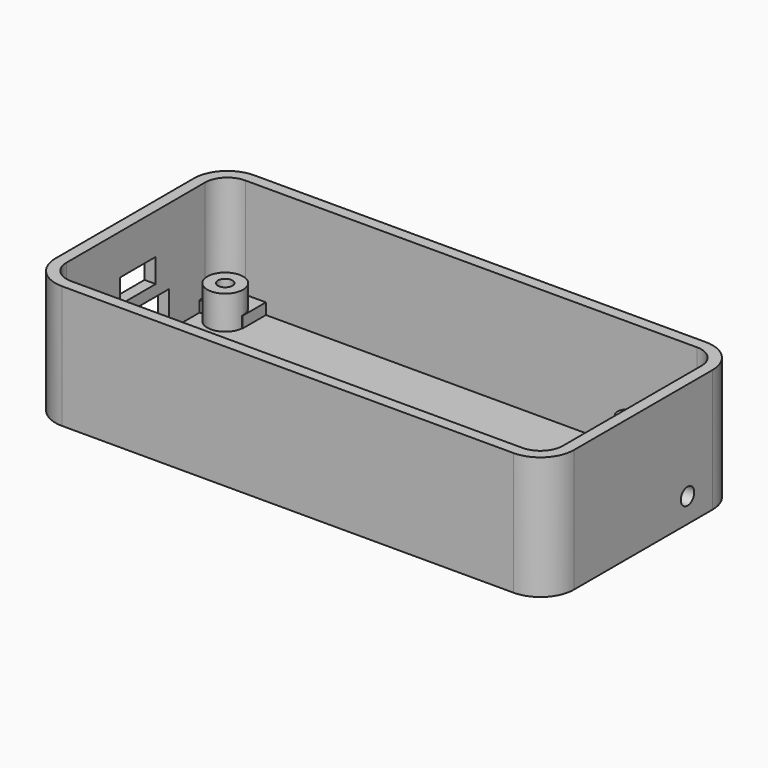
from build123d import *

# Parameters (mm, degrees)
F1_DEPTH  = 13.97
F2_T      = -1.27
F3_R      = 2.032
F3_R_2    = 0.8255
F4_DEPTH  = 3.81
F5_DEPTH  = 5.461
F6_DEPTH  = 2.54
F7_W      = 8.89
F7_H      = 3.1753103511
F7_W_2    = 5.08
F7_H_2    = 2.7178
F8_DEPTH  = 1.905
F9_R      = 0.9525
F10_DEPTH = 1.905
F11_R     = 2.032
F11_R_2   = 0.8255
F12_DEPTH = 3.81
F14_DEPTH = 2.032
F15_W     = 3.3083129674
F15_H     = 4.001185298
F15_W_2   = 4.9948431551
F15_H_2   = 3.4223934636
F15_W_3   = 4.9023460597
F15_H_3   = 4.0236227214
F16_DEPTH = 1.27


with BuildPart() as f1:
    # F0 (on Top) → F1 (new body)
    with BuildSketch(Plane.XY):
        with BuildLine():
            Line((-21.5788040441, -13.9683183577), (29.7179990722, -13.9683183577))
            ThreePointArc((29.7179990722, -13.9683183577), (32.4120759085, -12.852395194), (33.5279990722, -10.1583183577))
            Line((33.5279990722, -10.1583183577), (33.5279990722, 9.5266816423))
            ThreePointArc((33.5279990722, 9.5266816423), (32.4120759085, 12.2207584786), (29.7179990722, 13.3366816423))
            Line((29.7179990722, 13.3366816423), (-21.60052527, 13.3366816423))
            ThreePointArc((-21.60052527, 13.3366816423), (-24.2960880723, 12.2192716925), (-25.4105229505, 9.5224775366))
            Line((-25.4105229505, 9.5224775366), (-25.3888017246, -10.1625224634))
            ThreePointArc((-25.3888017246, -10.1625224634), (-24.2713940943, -12.8538811601), (-21.5788040441, -13.9683183577))
        make_face()
    extrude(amount=F1_DEPTH)

    # F2
    f2_openings = [f1.faces().sort_by_distance(p)[0] for p in [
        (4.064166, -0.31477, 13.97),
    ]]
    offset(amount=F2_T, openings=f2_openings)

    # F3 (on face) → F4 (join)
    with BuildSketch(Plane.XY.offset(1.27)):
        with Locations((-21.3360009278, 8.8916816423)):
            Circle(F3_R)
        with Locations((-21.3360009278, 8.8916816423)):
            Circle(F3_R_2, mode=Mode.SUBTRACT)
        with Locations((-21.3360009278, -8.8883183577)):
            Circle(F3_R)
        with Locations((-21.3360009278, -8.8883183577)):
            Circle(F3_R_2, mode=Mode.SUBTRACT)
        with BuildLine():
            Line((26.9239990722, -8.8883183577), (25.5269990722, -8.8883183577))
            ThreePointArc((25.5269990722, -8.8883183577), (24.3839990722, -10.0313183577), (23.2409990722, -8.8883183577))
            Line((23.2409990722, -8.8883183577), (21.8439990722, -8.8883183577))
            ThreePointArc((21.8439990722, -8.8883183577), (24.3839990722, -11.4283183577), (26.9239990722, -8.8883183577))
        make_face()
        with BuildLine():
            ThreePointArc((23.2409990722, 8.8916816423), (24.3839990722, 10.0346816423), (25.5269990722, 8.8916816423))
            Line((25.5269990722, 8.8916816423), (26.9239990722, 8.8916816423))
            ThreePointArc((26.9239990722, 8.8916816423), (24.3839990722, 11.4316816423), (21.8439990722, 8.8916816423))
            Line((21.8439990722, 8.8916816423), (23.2409990722, 8.8916816423))
        make_face()
    extrude(amount=F4_DEPTH)

    # F3 (on face) → F5 (join)
    with BuildSketch(Plane.XY.offset(1.27)):
        with BuildLine():
            Line((24.3839990722, 8.8916816423), (25.5269990722, 8.8916816423))
            ThreePointArc((25.5269990722, 8.8916816423), (24.3839990722, 10.0346816423), (23.2409990722, 8.8916816423))
            Line((23.2409990722, 8.8916816423), (24.3839990722, 8.8916816423))
        make_face()
        with BuildLine():
            ThreePointArc((23.2409990722, 8.8916816423), (24.3839990722, 7.7486816423), (25.5269990722, 8.8916816423))
            Line((25.5269990722, 8.8916816423), (24.3839990722, 8.8916816423))
            Line((24.3839990722, 8.8916816423), (23.2409990722, 8.8916816423))
        make_face()
        with BuildLine():
            Line((24.3839990722, -8.8883183577), (25.5269990722, -8.8883183577))
            ThreePointArc((25.5269990722, -8.8883183577), (24.3839990722, -7.7453183577), (23.2409990722, -8.8883183577))
            Line((23.2409990722, -8.8883183577), (24.3839990722, -8.8883183577))
        make_face()
        with BuildLine():
            ThreePointArc((23.2409990722, -8.8883183577), (24.3839990722, -10.0313183577), (25.5269990722, -8.8883183577))
            Line((25.5269990722, -8.8883183577), (24.3839990722, -8.8883183577))
            Line((24.3839990722, -8.8883183577), (23.2409990722, -8.8883183577))
        make_face()
    extrude(amount=F5_DEPTH)

    # F3 (on face) → F6 (cut)
    with BuildSketch(Plane.XY.offset(1.27)):
        with Locations((-21.3360009278, 8.8916816423)):
            Circle(F3_R_2)
        with Locations((-21.3360009278, -8.8883183577)):
            Circle(F3_R_2)
    extrude(amount=F6_DEPTH, mode=Mode.SUBTRACT)

    # F7 (on face) → F8 (cut)
    with BuildSketch(Plane(origin=(-25.3999845367, -0.0280273712, 0), x_dir=(0.0011034398, -0.9999993912, 0), z_dir=(-0.9999993912, -0.0011034398, 0))):
        with Locations((0, 3.81)):
            Rectangle(F7_W, F7_H)
        with Locations((0, 8.0265551756)):
            Rectangle(F7_W_2, F7_H_2)
    extrude(amount=-F8_DEPTH, mode=Mode.SUBTRACT)

    # F9 (on face) → F10 (cut)
    with BuildSketch(Plane.YZ.offset(33.5279990722)):
        with Locations((5.9706816423, 2.794)):
            Circle(F9_R)
    extrude(amount=-F10_DEPTH, mode=Mode.SUBTRACT)

    # F11 (on face) → F12 (join)
    with BuildSketch(Plane.XY.offset(1.27)):
        with Locations((29.4639990722, 0)):
            Circle(F11_R)
        with Locations((29.4639990722, 0)):
            Circle(F11_R_2, mode=Mode.SUBTRACT)
    extrude(amount=F12_DEPTH)

    # F13 (on face) → F14 (join)
    with BuildSketch(Plane.XY.offset(1.27)):
        with BuildLine():
            ThreePointArc((-14.0236731965, -12.6983183577), (-16.3756129487, -11.7037291087), (-17.9839668508, -9.7202911598))
            Line((-17.9839668508, -9.7202911598), (-18.9684356708, -10.3109590834))
            ThreePointArc((-18.9684356708, -10.3109590834), (-18.1080100407, -11.6293001054), (-16.9523477667, -12.6983183577))
            Line((-16.9523477667, -12.6983183577), (-14.0236731965, -12.6983183577))
        make_face()
        with BuildLine():
            ThreePointArc((-12.3923286591, -12.6983183577), (-13.2080009278, -12.7618183577), (-14.0236731965, -12.6983183577))
            Line((-14.0236731965, -12.6983183577), (-16.9523477667, -12.6983183577))
            ThreePointArc((-16.9523477667, -12.6983183577), (-13.2080009278, -13.9048183577), (-9.4636540889, -12.6983183577))
            Line((-9.4636540889, -12.6983183577), (-12.3923286591, -12.6983183577))
        make_face()
        with BuildLine():
            ThreePointArc((-16.6064980594, -3.4628710766), (-8.4130955389, -5.303384958), (-12.3923286591, -12.6983183577))
            Line((-12.3923286591, -12.6983183577), (-9.4636540889, -12.6983183577))
            ThreePointArc((-9.4636540889, -12.6983183577), (-8.145657173, -3.5535959249), (-17.3335159362, -2.5808083877))
            Line((-17.3335159362, -2.5808083877), (-16.6064980594, -3.4628710766))
        make_face()
    extrude(amount=F14_DEPTH)

    # F15 (on face) → F16 (join)
    with BuildSketch(Plane.XY.offset(1.27)):
        with Locations((31.0986405239, -0.0055211131)):
            Rectangle(F15_W, F15_H)
        with Locations((-21.7511262745, 10.4752979241)):
            Rectangle(F15_W_2, F15_H_2)
        with Locations((-21.7973748222, -10.8221620321)):
            Rectangle(F15_W_3, F15_H_3)
    extrude(amount=F16_DEPTH)


solid = f1.part
